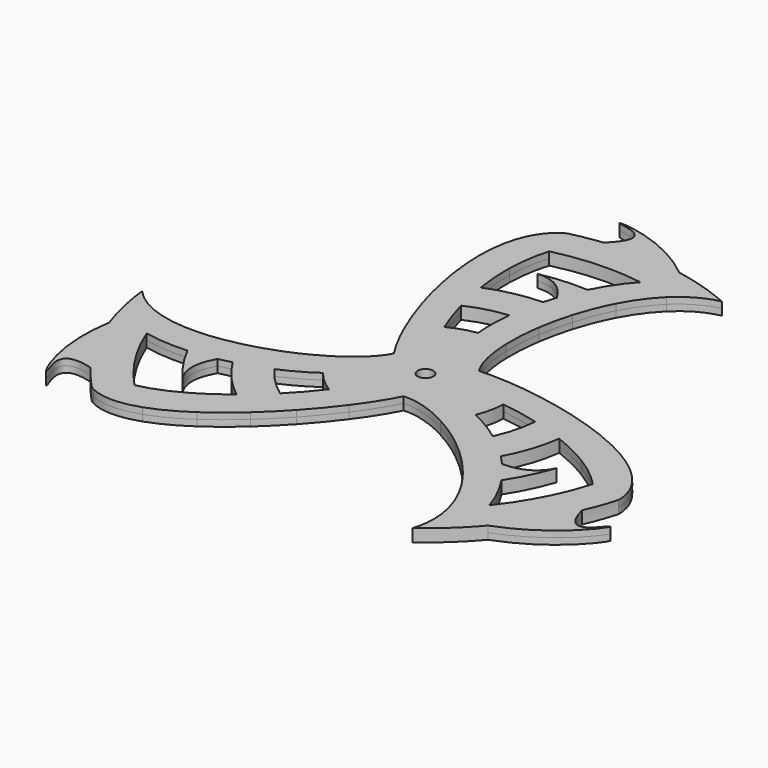
from build123d import *

# Parameters (mm, degrees)
F0_R     = 2.3749
F1_DEPTH = 1.905
F2_COUNT = 3
F3_R     = 5.08


# Not quite as in the source:
# - a feature names something its author has since deleted; it is built from what else it names


with BuildPart() as f1:
    # F0 (on Top) → F1 (new body, symmetric)
    with BuildSketch(Plane.XY):
        with BuildLine():
            ThreePointArc((-17.3653660324, 42.6367853949), (-21.7540823718, 40.5735296272), (-25.9014110749, 38.0600618835))
            add(Edge.make_bspline(
                [(-23.0965353089, 27.4544179136), (-24.1804087511, 30.9195032707), (-25.1340284277, 34.4901273217), (-25.9014110749, 38.0600618835)],
                knots=[24.4488898987, 24.4488898987, 24.4488898987, 24.4488898987, 33.2587639794, 33.2587639794, 33.2587639794, 33.2587639794], degree=3))
            ThreePointArc((-23.0965353089, 27.4544179136), (-19.3255134354, 30.2277941092), (-15.2255088291, 32.4865954995))
            add(Edge.make_bspline(
                [(-15.2255088291, 32.4865954995), (-16.1178743117, 35.7726004305), (-16.8502521039, 39.1913478949), (-17.3653660324, 42.6367853949)],
                knots=[23.1318038809, 23.1318038809, 23.1318038809, 23.1318038809, 31.9267236898, 31.9267236898, 31.9267236898, 31.9267236898], degree=3))
        make_face()
        with BuildLine():
            ThreePointArc((-16.2748742161, 67.2743985053), (-21.813442503, 65.6878219396), (-27.2008741383, 63.6461206289))
            add(Edge.make_bspline(
                [(-27.7469978607, 50.5063243444), (-28.0921321557, 55.2175644151), (-27.9588419563, 59.6900015587), (-27.2008741383, 63.6461206289)],
                knots=[43.6424910217, 43.6424910217, 43.6424910217, 43.6424910217, 55.7759701416, 55.7759701416, 55.7759701416, 55.7759701416], degree=3))
            ThreePointArc((-27.7469978607, 50.5063243444), (-23.0627332659, 52.8099898065), (-18.1892238673, 54.6803147775))
            add(Edge.make_bspline(
                [(-18.1892238673, 54.6803147775), (-18.0935641949, 59.1311544944), (-17.4997253093, 63.411166878), (-16.2748742161, 67.2743985053)],
                knots=[42.2257517636, 42.2257517636, 42.2257517636, 42.2257517636, 53.8672588581, 53.8672588581, 53.8672588581, 53.8672588581], degree=3))
        make_face()
        with BuildLine():
            ThreePointArc((-9.0210541083, 78.8607076292), (-14.0496453204, 78.1216877146), (-19.0206301357, 77.0623530282))
            add(Edge.make_bspline(
                [(-27.2008741383, 63.6461206289), (-26.0588797807, 69.6066186191), (-23.4988655122, 74.3950731638), (-19.0206301357, 77.0623530282)],
                knots=[55.7759701416, 55.7759701416, 55.7759701416, 55.7759701416, 74.0569107869, 74.0569107869, 74.0569107869, 74.0569107869], degree=3))
            ThreePointArc((-27.2008741383, 63.6461206289), (-21.813442503, 65.6878219396), (-16.2748742161, 67.2743985053))
            add(Edge.make_bspline(
                [(-16.2748742161, 67.2743985053), (-14.820591656, 71.8612665846), (-12.476762371, 75.8605930089), (-9.0210541083, 78.8607076292)],
                knots=[53.8672588581, 53.8672588581, 53.8672588581, 53.8672588581, 67.6893804491, 67.6893804491, 67.6893804491, 67.6893804491], degree=3))
        make_face()
        with BuildLine():
            ThreePointArc((12.7, 0), (11.8226431354, 4.6384382386), (9.3117938122, 8.636))
            ThreePointArc((9.3117938122, 8.636), (5.08, 11.6397422652), (0, 12.7))
            ThreePointArc((0, 12.7), (-3.0416717805, 12.3303784524), (-5.9062935719, 11.2430287842))
            ThreePointArc((-5.9062935719, 11.2430287842), (-9.9104189877, 7.94188866), (-12.2598045, 3.314693594))
            ThreePointArc((-12.2598045, 3.314693594), (-1.6718975522, -12.5894701467), (12.7, 0))
        make_face()
        Circle(F0_R, mode=Mode.SUBTRACT)
        with BuildLine():
            add(Edge.make_bspline(
                [(14.6040271988, 78.0199526697), (0, 90.0992277434), (-24.9292067048, 89.3250926774), (0, 87.5961761219), (-9.0210541083, 78.8607076292)],
                knots=[0, 0, 0, 0, 0.6246873254, 1, 1, 1, 1], degree=3))
            ThreePointArc((-9.0210541083, 78.8607076292), (2.8229619831, 79.3247849707), (14.6040271988, 78.0199526697))
        make_face()
        with BuildLine():
            add(Edge.make_bspline(
                [(10.4704118813, 68.4184675364), (13.8283543645, 72.0556456867), (17.7494139446, 74.8104964439), (22.1896866695, 76.2102908439)],
                knots=[53.8130004554, 53.8130004554, 53.8130004554, 53.8130004554, 67.275101171, 67.275101171, 67.275101171, 67.275101171], degree=3))
            ThreePointArc((22.1896866695, 76.2102908439), (18.4190950928, 77.2083386751), (14.6040271988, 78.0199526697))
            ThreePointArc((14.6040271988, 78.0199526697), (2.8229619831, 79.3247849707), (-9.0210541083, 78.8607076292))
            add(Edge.make_bspline(
                [(-16.2748742161, 67.2743985053), (-14.820591656, 71.8612665846), (-12.476762371, 75.8605930089), (-9.0210541083, 78.8607076292)],
                knots=[53.8672588581, 53.8672588581, 53.8672588581, 53.8672588581, 67.6893804491, 67.6893804491, 67.6893804491, 67.6893804491], degree=3))
            ThreePointArc((-16.2748742161, 67.2743985053), (-2.9580684975, 69.151761046), (10.4704118813, 68.4184675364))
        make_face()
        with BuildLine():
            add(Edge.make_bspline(
                [(20.0587079992, 66.244731552), (23.3867749165, 69.5042272729), (27.282013154, 71.829092762), (31.7428274143, 72.7515191095)],
                knots=[55.3953983219, 55.3953983219, 55.3953983219, 55.3953983219, 67.926070541, 67.926070541, 67.926070541, 67.926070541], degree=3))
            ThreePointArc((31.7428274143, 72.7515191096), (27.0216541745, 74.6339120687), (22.1896866695, 76.2102908439))
            add(Edge.make_bspline(
                [(10.4704118813, 68.4184675364), (13.8283543645, 72.0556456867), (17.7494139446, 74.8104964439), (22.1896866695, 76.2102908439)],
                knots=[53.8130004554, 53.8130004554, 53.8130004554, 53.8130004554, 67.275101171, 67.275101171, 67.275101171, 67.275101171], degree=3))
            ThreePointArc((10.4704118813, 68.4184675364), (15.3032046383, 67.5020603596), (20.0587079992, 66.244731552))
        make_face()
        with BuildLine():
            add(Edge.make_bspline(
                [(8.4234448453, 45.2603246032), (9.5576856112, 49.0741590808), (11.0162813262, 52.7833770574), (12.7985467127, 56.1870260034)],
                knots=[35.2826712732, 35.2826712732, 35.2826712732, 35.2826712732, 44.7374063862, 44.7374063862, 44.7374063862, 44.7374063862], degree=3))
            ThreePointArc((12.7985467127, 56.1870260034), (8.0098480092, 57.0668645006), (3.1639702107, 57.5393255224))
            add(Edge.make_bspline(
                [(0, 49.8570484138), (0.8932108743, 52.5016741843), (1.9498342067, 55.0836082307), (3.1639702107, 57.5393255224)],
                knots=[35.4915037863, 35.4915037863, 35.4915037863, 35.4915037863, 42.3868655915, 42.3868655915, 42.3868655915, 42.3868655915], degree=3))
            add(Edge.make_bspline(
                [(-1.1698454765, 46.0226342989), (-0.8177816603, 47.3104940467), (-0.4276173842, 48.5909555048), (0, 49.8570484138)],
                knots=[32.190405845, 32.190405845, 32.190405845, 32.190405845, 35.4915037863, 35.4915037863, 35.4915037863, 35.4915037863], degree=3))
            ThreePointArc((-1.1698454765, 46.0226342989), (3.646773227, 45.8928366009), (8.4234448453, 45.2603246032))
        make_face()
        with BuildLine():
            add(Edge.make_bspline(
                [(6.2199019454, 35.3342302313), (6.7150994299, 38.6352728385), (7.4497582363, 41.9863463866), (8.4234448453, 45.2603246032)],
                knots=[27.1662737248, 27.1662737248, 27.1662737248, 27.1662737248, 35.2826712732, 35.2826712732, 35.2826712732, 35.2826712732], degree=3))
            ThreePointArc((8.4234448453, 45.2603246032), (3.646773227, 45.8928366009), (-1.1698454765, 46.0226342989))
            add(Edge.make_bspline(
                [(-3.1562541704, 35.7383976398), (-2.7707896707, 39.1316542711), (-2.1046144953, 42.6032218584), (-1.1698454765, 46.0226342989)],
                knots=[23.4256196274, 23.4256196274, 23.4256196274, 23.4256196274, 32.190405845, 32.190405845, 32.190405845, 32.190405845], degree=3))
            ThreePointArc((-3.1562541704, 35.7383976398), (1.5450961931, 35.8442140938), (6.2199019454, 35.3342302313))
        make_face()
        with BuildLine():
            add(Edge.make_bspline(
                [(9.3117938122, 8.636), (6.9505323323, 11.9082742787), (5.6742637238, 17.3222002955), (5.4788445549, 23.6627479153)],
                knots=[0, 0, 0, 0, 17.2245237688, 17.2245237688, 17.2245237688, 17.2245237688], degree=3))
            ThreePointArc((5.4788445549, 23.6627479153), (1.1037248349, 24.2636594118), (-3.3078826047, 24.0624456204))
            add(Edge.make_bspline(
                [(-2.378855015, 18.6991668817), (-2.8065772797, 20.3730474275), (-3.1152579401, 22.1715226984), (-3.3078826047, 24.0624456204)],
                knots=[7.3898051274, 7.3898051274, 7.3898051274, 7.3898051274, 12.8846560588, 12.8846560588, 12.8846560588, 12.8846560588], degree=3))
            add(Edge.make_bspline(
                [(0, 12.7), (-1.0130974961, 14.4222450056), (-1.8036284575, 16.4480319202), (-2.378855015, 18.6991668817)],
                knots=[0, 0, 0, 0, 7.3898051274, 7.3898051274, 7.3898051274, 7.3898051274], degree=3))
            ThreePointArc((0, 12.7), (5.08, 11.6397422652), (9.3117938122, 8.636))
        make_face()
        with BuildLine():
            add(Edge.make_bspline(
                [(-3.1562541704, 35.7383976398), (-2.7707896707, 39.1316542711), (-2.1046144953, 42.6032218584), (-1.1698454765, 46.0226342989)],
                knots=[23.4256196274, 23.4256196274, 23.4256196274, 23.4256196274, 32.190405845, 32.190405845, 32.190405845, 32.190405845], degree=3))
            ThreePointArc((-1.1698454765, 46.0226342989), (-9.4209611835, 45.0632543946), (-17.3653660324, 42.6367853949))
            add(Edge.make_bspline(
                [(-15.2255088291, 32.4865954995), (-16.1178743117, 35.7726004305), (-16.8502521039, 39.1913478949), (-17.3653660324, 42.6367853949)],
                knots=[23.1318038809, 23.1318038809, 23.1318038809, 23.1318038809, 31.9267236898, 31.9267236898, 31.9267236898, 31.9267236898], degree=3))
            ThreePointArc((-15.2255088291, 32.4865954995), (-9.3335875756, 34.6421585531), (-3.1562541704, 35.7383976398))
        make_face()
        with BuildLine():
            ThreePointArc((-18.1892238673, 54.6803147775), (-23.0627332659, 52.8099898065), (-27.7469978607, 50.5063243444))
            add(Edge.make_bspline(
                [(-25.9014110749, 38.0600618835), (-26.8058839282, 42.2677526756), (-27.4516349004, 46.4744856243), (-27.7469978607, 50.5063243444)],
                knots=[33.2587639794, 33.2587639794, 33.2587639794, 33.2587639794, 43.6424910217, 43.6424910217, 43.6424910217, 43.6424910217], degree=3))
            ThreePointArc((-25.9014110749, 38.0600618835), (-21.7540823718, 40.5735296272), (-17.3653660324, 42.6367853949))
            add(Edge.make_bspline(
                [(-17.3653660324, 42.6367853949), (-17.9685748082, 46.6714620389), (-18.2738522272, 50.7427384119), (-18.1892238673, 54.6803147775)],
                knots=[31.9267236898, 31.9267236898, 31.9267236898, 31.9267236898, 42.2257517636, 42.2257517636, 42.2257517636, 42.2257517636], degree=3))
        make_face()
        with BuildLine():
            add(Edge.make_bspline(
                [(12.7985467127, 56.1870260034), (14.8076320957, 60.0238403176), (17.2280130656, 63.4723600065), (20.0587079992, 66.244731552)],
                knots=[44.7374063862, 44.7374063862, 44.7374063862, 44.7374063862, 55.3953983219, 55.3953983219, 55.3953983219, 55.3953983219], degree=3))
            ThreePointArc((20.0587079992, 66.244731552), (15.3032046383, 67.5020603596), (10.4704118813, 68.4184675364))
            add(Edge.make_bspline(
                [(3.1639702107, 57.5393255224), (5.1758851932, 61.6086343933), (7.6203140781, 65.3313647918), (10.4704118813, 68.4184675364)],
                knots=[42.3868655915, 42.3868655915, 42.3868655915, 42.3868655915, 53.8130004554, 53.8130004554, 53.8130004554, 53.8130004554], degree=3))
            ThreePointArc((3.1639702107, 57.5393255224), (8.0098480092, 57.0668645006), (12.7985467127, 56.1870260034))
        make_face()
        with BuildLine():
            add(Edge.make_bspline(
                [(0, 49.8570484138), (0.8932108743, 52.5016741843), (1.9498342067, 55.0836082307), (3.1639702107, 57.5393255224)],
                knots=[35.4915037863, 35.4915037863, 35.4915037863, 35.4915037863, 42.3868655915, 42.3868655915, 42.3868655915, 42.3868655915], degree=3))
            ThreePointArc((3.1639702107, 57.5393255224), (-4.0756357354, 57.4819439686), (-11.2509119437, 56.5172687725))
            add(Edge.make_bspline(
                [(0, 49.8570484138), (-1.1688542807, 51.7104393634), (-4.3519753437, 57.0861568163), (-11.2509119437, 56.5172687725)],
                knots=[0, 0, 0, 0, 13.0744619312, 13.0744619312, 13.0744619312, 13.0744619312], degree=3))
        make_face()
        with BuildLine():
            ThreePointArc((-14.9722977082, 19.1252105322), (-16.9249939283, 17.4209057483), (-18.6849654693, 15.518229344))
            add(Edge.make_bspline(
                [(-12.2598045, 3.314693594), (-14.411503383, 6.5386225656), (-16.6246307846, 10.7419626704), (-18.6849654693, 15.518229344)],
                knots=[0, 0, 0, 0, 13.7796378213, 13.7796378213, 13.7796378213, 13.7796378213], degree=3))
            ThreePointArc((-12.2598045, 3.314693594), (-9.9104189877, 7.94188866), (-5.9062935719, 11.2430287842))
            add(Edge.make_bspline(
                [(-5.9062935719, 11.2430287842), (-7.6243659406, 13.6243057921), (-9.3270259787, 16.684630565), (-10.8929366742, 20.1993356284)],
                knots=[0, 0, 0, 0, 11.2954876408, 11.2954876408, 11.2954876408, 11.2954876408], degree=3))
            add(Edge.make_bspline(
                [(-10.8929366742, 20.1993356284), (-12.1686662763, 20.0425592524), (-13.5369923905, 19.7089447328), (-14.9722977082, 19.1252105322)],
                knots=[9.572986719, 9.572986719, 9.572986719, 9.572986719, 12.6006472873, 12.6006472873, 12.6006472873, 12.6006472873], degree=3))
        make_face()
        with BuildLine():
            add(Edge.make_bspline(
                [(5.4788445549, 23.6627479153), (5.3660513921, 27.3224217541), (5.6133360964, 31.2907934727), (6.2199019454, 35.3342302313)],
                knots=[17.2245237688, 17.2245237688, 17.2245237688, 17.2245237688, 27.1662737248, 27.1662737248, 27.1662737248, 27.1662737248], degree=3))
            ThreePointArc((6.2199019454, 35.3342302313), (1.5450961931, 35.8442140938), (-3.1562541704, 35.7383976398))
            add(Edge.make_bspline(
                [(-3.3078826047, 24.0624456204), (-3.6774011954, 27.6898687991), (-3.6198327617, 31.657500098), (-3.1562541704, 35.7383976398)],
                knots=[12.8846560588, 12.8846560588, 12.8846560588, 12.8846560588, 23.4256196274, 23.4256196274, 23.4256196274, 23.4256196274], degree=3))
            ThreePointArc((-3.3078826047, 24.0624456204), (1.1037248349, 24.2636594118), (5.4788445549, 23.6627479153))
        make_face()
        with BuildLine():
            add(Edge.make_bspline(
                [(-10.8929366742, 20.1993356284), (-11.0733640979, 20.6043071133), (-11.2519760211, 21.0153110047), (-11.4285868345, 21.4320036284)],
                knots=[11.2954876408, 11.2954876408, 11.2954876408, 11.2954876408, 12.5969767614, 12.5969767614, 12.5969767614, 12.5969767614], degree=3))
            ThreePointArc((-11.4285868345, 21.4320036284), (-13.2507358194, 20.3558683629), (-14.9722977082, 19.1252105322))
            add(Edge.make_bspline(
                [(-10.8929366742, 20.1993356284), (-12.1686662763, 20.0425592524), (-13.5369923905, 19.7089447328), (-14.9722977082, 19.1252105322)],
                knots=[9.572986719, 9.572986719, 9.572986719, 9.572986719, 12.6006472873, 12.6006472873, 12.6006472873, 12.6006472873], degree=3))
        make_face()
        with BuildLine():
            ThreePointArc((-15.2255088291, 32.4865954995), (-19.3255134354, 30.2277941092), (-23.0965353089, 27.4544179136))
            add(Edge.make_bspline(
                [(-18.6849654693, 15.518229344), (-20.2802345469, 19.216381196), (-21.7839037243, 23.2580050244), (-23.0965353089, 27.4544179136)],
                knots=[13.7796378213, 13.7796378213, 13.7796378213, 13.7796378213, 24.4488898987, 24.4488898987, 24.4488898987, 24.4488898987], degree=3))
            ThreePointArc((-18.6849654693, 15.518229344), (-16.9249939283, 17.4209057483), (-14.9722977082, 19.1252105322))
            ThreePointArc((-14.9722977082, 19.1252105322), (-13.2507358194, 20.3558683629), (-11.4285868345, 21.4320036284))
            add(Edge.make_bspline(
                [(-11.4285868345, 21.4320036284), (-12.8581526731, 24.8048975568), (-14.1566058384, 28.5505171026), (-15.2255088291, 32.4865954995)],
                knots=[12.5969767614, 12.5969767614, 12.5969767614, 12.5969767614, 23.1318038809, 23.1318038809, 23.1318038809, 23.1318038809], degree=3))
        make_face()
        with BuildLine():
            add(Edge.make_bspline(
                [(-2.378855015, 18.6991668817), (-2.8065772797, 20.3730474275), (-3.1152579401, 22.1715226984), (-3.3078826047, 24.0624456204)],
                knots=[7.3898051274, 7.3898051274, 7.3898051274, 7.3898051274, 12.8846560588, 12.8846560588, 12.8846560588, 12.8846560588], degree=3))
            ThreePointArc((-3.3078826047, 24.0624456204), (-7.484696998, 23.1067671346), (-11.4285868345, 21.4320036284))
            add(Edge.make_bspline(
                [(-10.8929366742, 20.1993356284), (-11.0733640979, 20.6043071133), (-11.2519760211, 21.0153110047), (-11.4285868345, 21.4320036284)],
                knots=[11.2954876408, 11.2954876408, 11.2954876408, 11.2954876408, 12.5969767614, 12.5969767614, 12.5969767614, 12.5969767614], degree=3))
            add(Edge.make_bspline(
                [(-2.378855015, 18.6991668817), (-3.7513342636, 19.4228450426), (-6.8592802382, 20.6950378817), (-10.8929366742, 20.1993356284)],
                knots=[0, 0, 0, 0, 9.572986719, 9.572986719, 9.572986719, 9.572986719], degree=3))
        make_face()
        with BuildLine():
            ThreePointArc((-5.9062935719, 11.2430287842), (-3.0416717805, 12.3303784524), (0, 12.7))
            add(Edge.make_bspline(
                [(0, 12.7), (-1.0130974961, 14.4222450056), (-1.8036284575, 16.4480319202), (-2.378855015, 18.6991668817)],
                knots=[0, 0, 0, 0, 7.3898051274, 7.3898051274, 7.3898051274, 7.3898051274], degree=3))
            add(Edge.make_bspline(
                [(-2.378855015, 18.6991668817), (-3.7513342636, 19.4228450426), (-6.8592802382, 20.6950378817), (-10.8929366742, 20.1993356284)],
                knots=[0, 0, 0, 0, 9.572986719, 9.572986719, 9.572986719, 9.572986719], degree=3))
            add(Edge.make_bspline(
                [(-5.9062935719, 11.2430287842), (-7.6243659406, 13.6243057921), (-9.3270259787, 16.684630565), (-10.8929366742, 20.1993356284)],
                knots=[0, 0, 0, 0, 11.2954876408, 11.2954876408, 11.2954876408, 11.2954876408], degree=3))
        make_face()
    extrude(amount=F1_DEPTH, both=True)

    # F2: F1 ×3 about axis
    f2_axis = Axis((0, 0, 1.905), (0, 0, 1))


with BuildPart() as f1_1:
    add(f1.part)
    for i in range(1, F2_COUNT):
        add(f1.part.rotate(f2_axis, i * 360 / F2_COUNT))

    # F3
    f3_edges = [f1_1.edges().sort_by_distance(p)[0] for p in [
        (-19.02063, 77.062353, 0.9525),
        (-19.02063, 77.062353, -0.9525),
        (-57.22764, -55.003525, -0.9525),
    ]]
    fillet(f3_edges, radius=F3_R)


solid = f1_1.part
